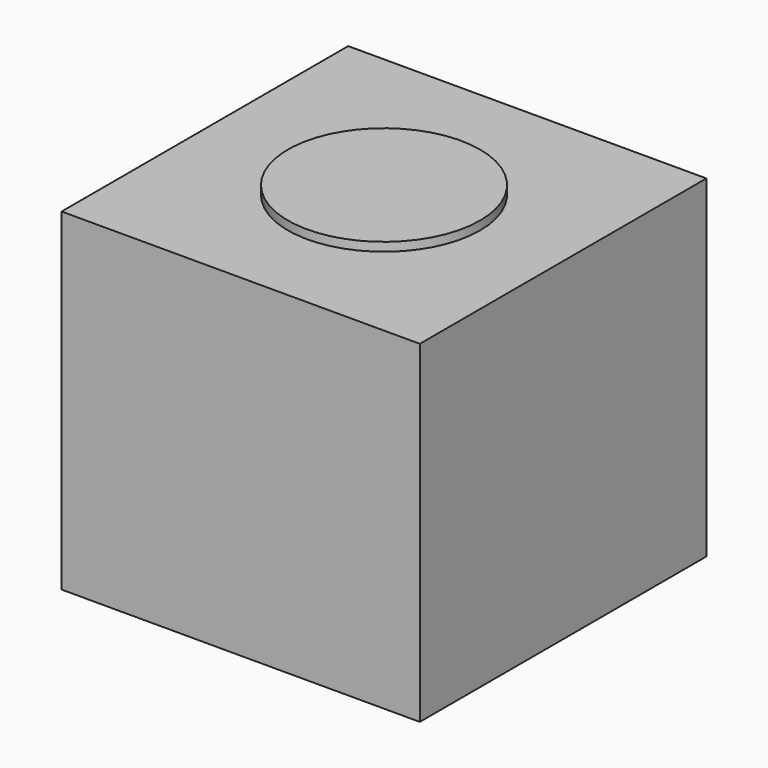
from build123d import *

# Parameters (mm, degrees)
F0_W     = 41
F0_H     = 41
F1_DEPTH = 38.1
F2_R     = 11
F3_DEPTH = 1


# Not quite as in the source:
# - the program builds the solid bodies; features that only make, move or delete a surface that nothing else refers to are left out


with BuildPart() as f1:
    # F0 (on Top) → F1 (new body)
    with BuildSketch(Plane.XY):
        Rectangle(F0_W, F0_H)
    extrude(amount=F1_DEPTH)

    # F2 (on face) → F3 (join)
    with BuildSketch(Plane.XY.offset(38.1)):
        Circle(F2_R)
    extrude(amount=F3_DEPTH)


solid = f1.part
